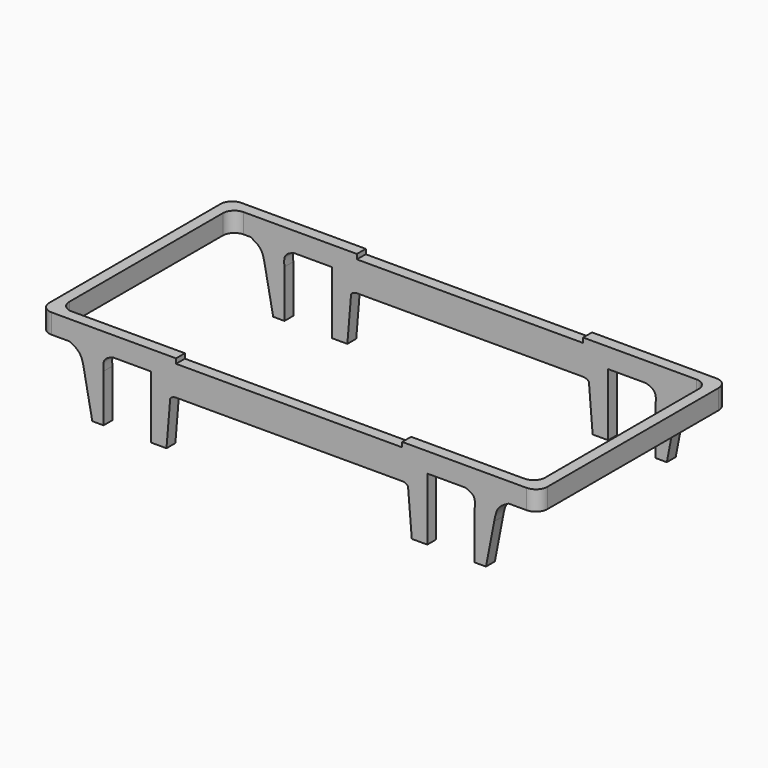
from build123d import *

# Parameters (mm, degrees)
F1_DEPTH = 12.192
F3_W     = 260.35
F3_H     = 21.6032387971
F4_DEPTH = 12.192
F5_W     = 260.35
F5_H     = 21.59
F6_DEPTH = 12.192
F7_R     = 12.7


with BuildPart() as f1:
    # F0 (on Front) → F1 (new body)
    with BuildSketch(Plane.XZ):
        Polygon((115.4489097687, 44.9104134451), (-8.7127741426, 44.9104134451), (-8.7127741426, 12.2448502547), (115.4489097687, 12.2448502547), (115.4489097687, 28.5776318499), align=None)
        with BuildLine():
            add(Edge.make_bspline(
                [(-201.3751125628, 28.5776318499), (-203.6036875056, 28.2155507261), (-213.5160050083, 24.8398299044), (-212.7768922816, 16.2961456434), (-212.3699930733, 11.8833564186)],
                knots=[0.1713367735, 0.1713367735, 0.1713367735, 0.1713367735, 0.5720981619, 1, 1, 1, 1], degree=3))
            Line((-201.3751125628, 28.5776318499), (-249.5887362649, 28.5776318499))
            add(Edge.make_bspline(
                [(-249.5887362649, 28.5776318499), (-245.3983662499, 26.3811930315), (-236.7722226078, 21.8596837899), (-234.7906912251, 11.49704289), (-233.7717394185, 6.1683199847)],
                knots=[0, 0, 0, 0, 0.4857755898, 1, 1, 1, 1], degree=3))
            Line((-233.7717394185, 6.1683199847), (-224.7518429065, -40.4246754655))
            Line((-224.7518429065, -40.4246754655), (-212.3699930733, -40.4246754655))
            Line((-212.3699930733, -40.4246754655), (-212.3699930733, 11.8833564186))
        make_face()
        with BuildLine():
            add(Edge.make_bspline(
                [(232.1631879797, 28.5776318499), (227.9728179646, 26.3811930315), (219.3466743226, 21.8596837899), (217.3651429399, 11.49704289), (216.3461911332, 6.1683199847)],
                knots=[0, 0, 0, 0, 0.4857755898, 1, 1, 1, 1], degree=3))
            Line((232.1631879797, 28.5776318499), (183.9495642776, 28.5776318499))
            add(Edge.make_bspline(
                [(183.9495642776, 28.5776318499), (186.1781392203, 28.2155507261), (196.0904567231, 24.8398299044), (195.3513439963, 16.2961456434), (194.944444788, 11.8833564186)],
                knots=[0.1713367735, 0.1713367735, 0.1713367735, 0.1713367735, 0.5720981619, 1, 1, 1, 1], degree=3))
            Line((194.944444788, 11.8833564186), (194.944444788, -40.4246754655))
            Line((194.944444788, -40.4246754655), (207.3262946213, -40.4246754655))
            Line((207.3262946213, -40.4246754655), (216.3461911332, 6.1683199847))
        make_face()
        with BuildLine():
            Line((-132.874458054, 12.2448502547), (-132.874458054, 28.5776318499))
            Line((-132.874458054, 28.5776318499), (-160.3592138582, 28.5776318499))
            Line((-160.3592138582, 28.5776318499), (-160.3592138582, -40.1182342476))
            Line((-160.3592138582, -40.1182342476), (-143.3239786863, -40.1182342476))
            Line((-143.3239786863, -40.1182342476), (-139.2062762381, 9.481767078))
            ThreePointArc((-139.2062762381, 9.481767078), (-136.3286783046, 11.5239959202), (-132.874458054, 12.2448502547))
        make_face()
        with BuildLine():
            Line((115.4489097687, 28.5776318499), (115.4489097687, 12.2448502547))
            ThreePointArc((115.4489097687, 12.2448502547), (118.9031300193, 11.5239959202), (121.7807279529, 9.481767078))
            Line((121.7807279529, 9.481767078), (125.898430401, -40.1182342476))
            Line((125.898430401, -40.1182342476), (142.933665573, -40.1182342476))
            Line((142.933665573, -40.1182342476), (142.933665573, 28.5776318499))
            Line((142.933665573, 28.5776318499), (115.4489097687, 28.5776318499))
        make_face()
        with BuildLine():
            Line((115.4489097687, 50.180870647), (115.4489097687, 44.9104134451))
            Line((115.4489097687, 44.9104134451), (115.4489097687, 28.5776318499))
            Line((115.4489097687, 28.5776318499), (142.933665573, 28.5776318499))
            Line((142.933665573, 28.5776318499), (182.0295738914, 28.5776318499))
            add(Edge.make_bspline(
                [(182.0295738914, 28.5776318499), (182.5128861487, 28.6550095059), (182.9967857635, 28.7324317216), (183.9495642776, 28.5776318499)],
                knots=[0, 0, 0, 0, 0.1713367735, 0.1713367735, 0.1713367735, 0.1713367735], degree=3))
            Line((183.9495642776, 28.5776318499), (232.1631879797, 28.5776318499))
            Line((232.1631879797, 28.5776318499), (252.4502187865, 28.5776318499))
            Line((252.4502187865, 28.5776318499), (252.4502187865, 50.180870647))
            Line((252.4502187865, 50.180870647), (115.4489097687, 50.180870647))
        make_face()
        Polygon((-8.7127741426, 44.9104134451), (-132.874458054, 44.9104134451), (-132.874458054, 28.5776318499), (-132.874458054, 12.2448502547), (-8.7127741426, 12.2448502547), align=None)
        with BuildLine():
            Line((-132.874458054, 28.5776318499), (-132.874458054, 44.9104134451))
            Line((-132.874458054, 44.9104134451), (-132.874458054, 50.180870647))
            Line((-132.874458054, 50.180870647), (-269.8757670717, 50.180870647))
            Line((-269.8757670717, 50.180870647), (-269.8757670717, 28.5776318499))
            Line((-269.8757670717, 28.5776318499), (-249.5887362649, 28.5776318499))
            Line((-249.5887362649, 28.5776318499), (-201.3751125628, 28.5776318499))
            add(Edge.make_bspline(
                [(-199.4551221767, 28.5776318499), (-199.9384344339, 28.6550095059), (-200.4223340487, 28.7324317216), (-201.3751125628, 28.5776318499)],
                knots=[0, 0, 0, 0, 0.1713367735, 0.1713367735, 0.1713367735, 0.1713367735], degree=3))
            Line((-199.4551221767, 28.5776318499), (-160.3592138582, 28.5776318499))
            Line((-160.3592138582, 28.5776318499), (-132.874458054, 28.5776318499))
        make_face()
        with BuildLine():
            add(Edge.make_bspline(
                [(182.0295738914, 28.5776318499), (182.5128861487, 28.6550095059), (182.9967857635, 28.7324317216), (183.9495642776, 28.5776318499)],
                knots=[0, 0, 0, 0, 0.1713367735, 0.1713367735, 0.1713367735, 0.1713367735], degree=3))
            Line((182.0295738914, 28.5776318499), (183.9495642776, 28.5776318499))
        make_face()
        with BuildLine():
            Line((-201.3751125628, 28.5776318499), (-199.4551221767, 28.5776318499))
            add(Edge.make_bspline(
                [(-199.4551221767, 28.5776318499), (-199.9384344339, 28.6550095059), (-200.4223340487, 28.7324317216), (-201.3751125628, 28.5776318499)],
                knots=[0, 0, 0, 0, 0.1713367735, 0.1713367735, 0.1713367735, 0.1713367735], degree=3))
        make_face()
    extrude(amount=F1_DEPTH)


with BuildPart() as f2_1:
    # F2: copy of F1
    add(f1.part.moved(Location((0, -248.158, 0))))


with BuildPart() as f1_1:
    add(f1.part)

    add(f2_1.part)  # F4 merges F2_1
    # F3 (on face) → F4 (join)
    with BuildSketch(Plane.YZ.offset(252.4502187865)):
        with Locations((-130.175, 39.3792512485)):
            Rectangle(F3_W, F3_H)
    extrude(amount=F4_DEPTH)

    # F5 (on face) → F6 (join)
    with BuildSketch(Plane(origin=(-269.8757670717, 0, 0), x_dir=(0, -1, 0), z_dir=(-1, 0, 0))):
        with Locations((130.175, 39.385870647)):
            Rectangle(F5_W, F5_H)
    extrude(amount=F6_DEPTH)

    # F7
    f7_edges = [f1_1.edges().sort_by_distance(p)[0] for p in [
        (264.642219, -260.35, 39.379251),
        (264.642219, 0, 39.379251),
        (-282.067767, 0, 39.385871),
        (-282.067767, -260.35, 39.385871),
        (252.450219, -12.192, 39.379251),
        (252.450219, -248.158, 39.379251),
        (-269.875767, -248.158, 39.385871),
        (-269.875767, -12.192, 39.385871),
    ]]
    fillet(f7_edges, radius=F7_R)


solid = f1_1.part
